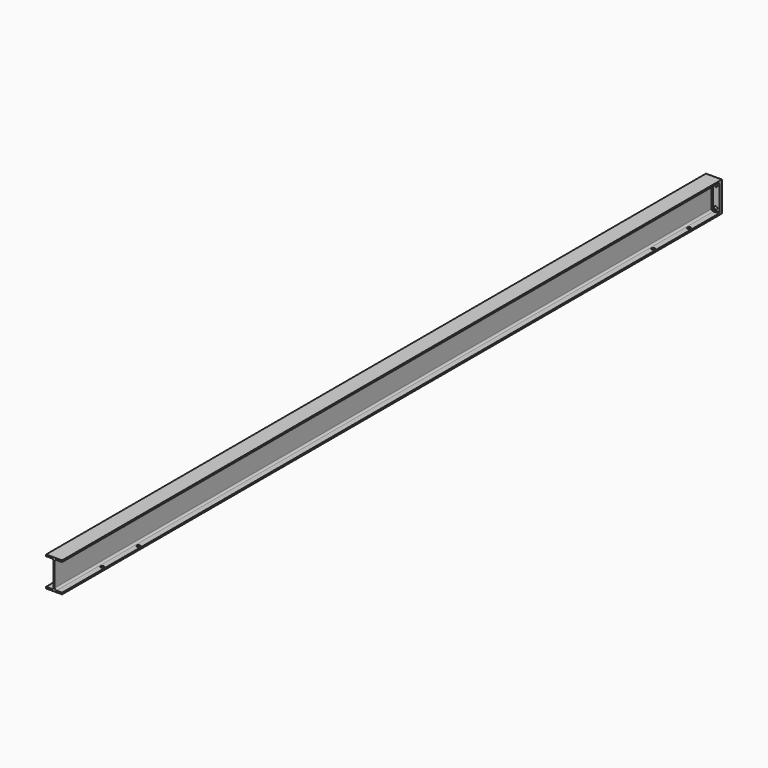
from build123d import *

# Parameters (mm, degrees)
F1_DEPTH      = 300
F1_DEPTH_BACK = 3000
F2_R          = 6.5
F3_DEPTH      = 12
F4_SIZE       = 3
F5_SIZE       = 3
F6_R          = 6.5
F7_DEPTH      = 6.3


# Not quite as in the source:
# - a feature names something its author has since deleted; it is built from what else it names


with BuildPart() as f1:
    # F0 (on Front) → F1 (new body, two sides)
    with BuildSketch(Plane.XZ) as f1_sk:
        with BuildLine():
            Line((-32, 6.3), (-32, 0))
            Line((-32, 0), (32, 0))
            Line((32, 0), (32, 6.3))
            Line((32, 6.3), (9.2, 6.3))
            ThreePointArc((9.2, 6.3), (4.2502525317, 8.3502525317), (2.2, 13.3))
            Line((2.2, 13.3), (2.2, 106.7))
            ThreePointArc((2.2, 106.7), (4.2502525317, 111.6497474683), (9.2, 113.7))
            Line((9.2, 113.7), (32, 113.7))
            Line((32, 113.7), (32, 120))
            Line((32, 120), (-32, 120))
            Line((-32, 120), (-32, 113.7))
            Line((-32, 113.7), (-9.2, 113.7))
            ThreePointArc((-9.2, 113.7), (-4.2502525317, 111.6497474683), (-2.2, 106.7))
            Line((-2.2, 106.7), (-2.2, 13.3))
            ThreePointArc((-2.2, 13.3), (-4.2502525317, 8.3502525317), (-9.2, 6.3))
            Line((-9.2, 6.3), (-32, 6.3))
        make_face()
    extrude(amount=F1_DEPTH)
    extrude(f1_sk.sketch, amount=-F1_DEPTH_BACK)

    # F2 (on face) → F3 (join)
    with BuildSketch(Plane(origin=(0, 3000, 0), x_dir=(-1, 0, 0), z_dir=(0, 1, 0))):
        with BuildLine():
            Line((9.2, 6.3), (32, 6.3))
            Line((32, 6.3), (32, 113.7))
            Line((32, 113.7), (9.2, 113.7))
            ThreePointArc((9.2, 113.7), (4.2502525317, 111.6497474683), (2.2, 106.7))
            Line((2.2, 106.7), (2.2, 13.3))
            ThreePointArc((2.2, 13.3), (4.2502525317, 8.3502525317), (9.2, 6.3))
        make_face()
        with Locations((17, 20)):
            Circle(F2_R, mode=Mode.SUBTRACT)
        with Locations((17, 100)):
            Circle(F2_R, mode=Mode.SUBTRACT)
        with BuildLine():
            Line((-32, 113.7), (-32, 6.3))
            Line((-32, 6.3), (-9.2, 6.3))
            ThreePointArc((-9.2, 6.3), (-4.2502525317, 8.3502525317), (-2.2, 13.3))
            Line((-2.2, 13.3), (-2.2, 106.7))
            ThreePointArc((-2.2, 106.7), (-4.2502525317, 111.6497474683), (-9.2, 113.7))
            Line((-9.2, 113.7), (-32, 113.7))
        make_face()
        with Locations((-17, 20)):
            Circle(F2_R, mode=Mode.SUBTRACT)
        with Locations((-17, 100)):
            Circle(F2_R, mode=Mode.SUBTRACT)
        with BuildLine():
            Line((-32, 6.3), (-32, 0))
            Line((-32, 0), (32, 0))
            Line((32, 0), (32, 6.3))
            Line((32, 6.3), (9.2, 6.3))
            ThreePointArc((9.2, 6.3), (4.2502525317, 8.3502525317), (2.2, 13.3))
            Line((2.2, 13.3), (2.2, 106.7))
            ThreePointArc((2.2, 106.7), (4.2502525317, 111.6497474683), (9.2, 113.7))
            Line((9.2, 113.7), (32, 113.7))
            Line((32, 113.7), (32, 120))
            Line((32, 120), (-32, 120))
            Line((-32, 120), (-32, 113.7))
            Line((-32, 113.7), (-9.2, 113.7))
            ThreePointArc((-9.2, 113.7), (-4.2502525317, 111.6497474683), (-2.2, 106.7))
            Line((-2.2, 106.7), (-2.2, 13.3))
            ThreePointArc((-2.2, 13.3), (-4.2502525317, 8.3502525317), (-9.2, 6.3))
            Line((-9.2, 6.3), (-32, 6.3))
        make_face()
    extrude(amount=-F3_DEPTH)

    # F4
    f4_edges = [f1.edges().sort_by_distance(p)[0] for p in [
        (20.6, 2988, 113.7),
        (4.250253, 2988, 111.649747),
        (2.2, 2988, 60),
        (4.250253, 2988, 8.350253),
        (20.6, 2988, 6.3),
    ]]
    chamfer(f4_edges, length=F4_SIZE)

    # F5
    f5_edges = [f1.edges().sort_by_distance(p)[0] for p in [
        (-20.6, 2988, 6.3),
        (-4.250253, 2988, 8.350253),
        (-2.2, 2988, 60),
        (-4.250253, 2988, 111.649747),
        (-20.6, 2988, 113.7),
    ]]
    chamfer(f5_edges, length=F5_SIZE)

    # F6 (on face) → F7 (cut, through all)
    with BuildSketch(Plane(origin=(0, 0, 0), x_dir=(1, 0, 0), z_dir=(0, 0, -1))):
        with Locations((21, 85)):
            Circle(F6_R)
        with Locations((-21, 85)):
            Circle(F6_R)
        with Locations((-21, -95)):
            Circle(F6_R)
        with Locations((21, -95)):
            Circle(F6_R)
        with Locations((-21, -2670)):
            Circle(F6_R)
        with Locations((21, -2670)):
            Circle(F6_R)
        with Locations((21, -2850)):
            Circle(F6_R)
        with Locations((-21, -2850)):
            Circle(F6_R)
    extrude(amount=-F7_DEPTH, mode=Mode.SUBTRACT)


solid = f1.part
